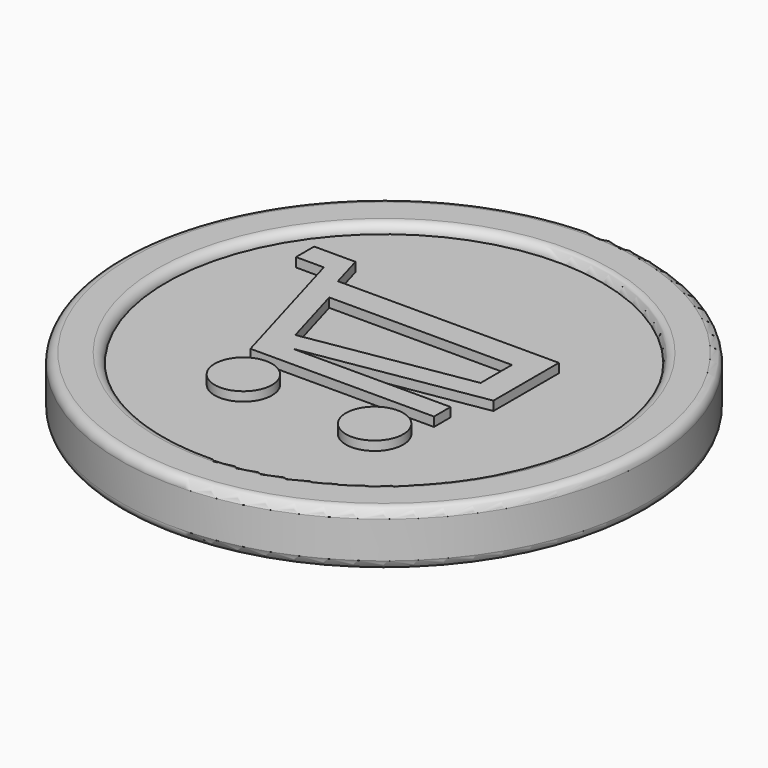
from build123d import *

# Parameters (mm, degrees)
F0_R     = 11.5
F1_DEPTH = 2
F2_R     = 11.5
F2_R_2   = 9.5
F3_DEPTH = 0.4
F4_R     = 1.25
F5_DEPTH = 0.4
F6_R     = 0.39999


# Not quite as in the source:
# - a fillet or chamfer is up to 0.001 mm smaller than in the source, because OpenCascade refuses the exact size


with BuildPart() as f1:
    # F0 (on Top) → F1 (new body)
    with BuildSketch(Plane.XY):
        Circle(F0_R)
    extrude(amount=F1_DEPTH)

    # F2 (on face) → F3 (join)
    with BuildSketch(Plane.XY.offset(2)):
        Circle(F2_R)
        Circle(F2_R_2, mode=Mode.SUBTRACT)
    extrude(amount=F3_DEPTH)

    # F4 (on face) → F5 (join)
    with BuildSketch(Plane.XY.offset(2)):
        Polygon((-4.9462847407, 4.6223603384), (-6.7446869929, 4.6223603384), (-6.7446869929, 3.631329312), (-5.5307656769, 3.631329312), (-3.7330235863, -2.611553217), (4.2630984261, -2.611553217), (4.2630984261, -1.7084874132), (-2.6016419292, -1.7084874132), (5.1088749777, -0.4323172916), (5.1088749777, 3.1326496529), (-4.5172977159, 3.1326496529), align=None)
        Polygon((-3.1724679652, -0.8662961763), (-4.0021237171, 2.0147863915), (3.9558067254, 2.0147863915), (3.9558067254, 0.3135068497), align=None, mode=Mode.SUBTRACT)
        with Locations((-2.7432420498, -4.2344009733)):
            Circle(F4_R)
        with Locations((3.0116447943, -4.2793590558)):
            Circle(F4_R)
    extrude(amount=F5_DEPTH)

    # F6 (radius 0.4 in the source; OpenCascade refuses exactly that, so slightly less here)
    f6_edges = [f1.edges().sort_by_distance(p)[0] for p in [
        (-11.5, 0, 2.4),
        (-9.5, 0, 2.4),
        (-11.5, 0, 0),
    ]]
    fillet(f6_edges, radius=F6_R)


solid = f1.part
